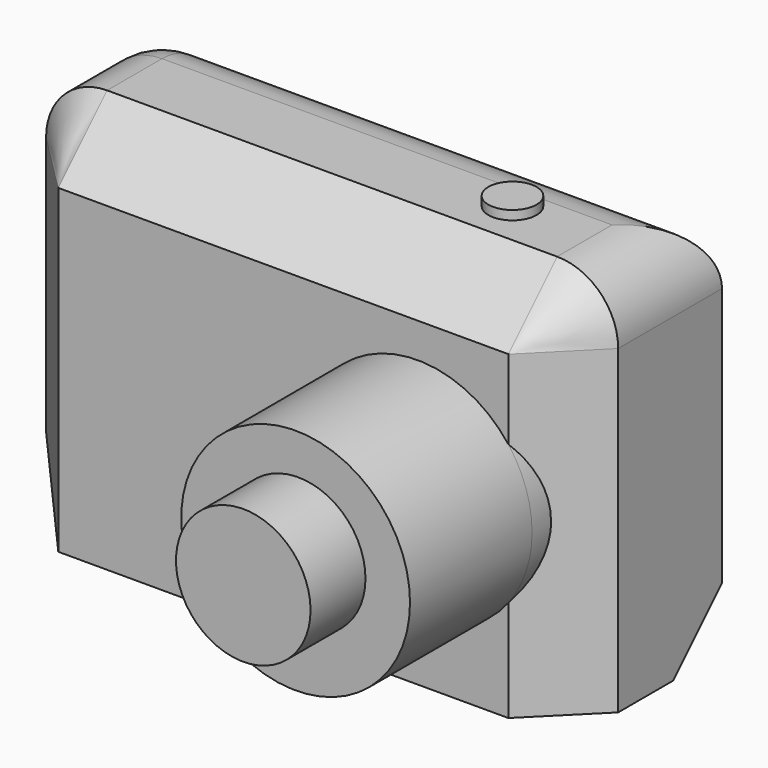
from build123d import *

# Parameters (mm, degrees)
F0_W         = 150
F0_H         = 50
F1_DEPTH     = 100
F2_R         = 30
F3_DEPTH     = 40
F4_R         = 16
F5_R         = 16
F6_T1_DEPTH  = 75.1469278075
F6_T3_DEPTH  = 125.1469278075
F6_T5_DEPTH  = 175.1469278075
F6_T7_DEPTH  = 118
F6_T10_ANGLE = 90
F6_T12_ANGLE = 90
F6_T14_ANGLE = 90
F6_T18_DEPTH = 125.1469278075
F6_S19_R     = 30
F6_T20_DEPTH = 65
F7_R         = 6.3155551437
F8_DEPTH     = 2.4
F9_R         = 17.6407421848
F10_DEPTH    = 18


# Not quite as in the source:
# - a fillet or chamfer that OpenCascade refuses, or shapes differently, is made with other operations: its cross-section is extruded or revolved along the edge and cut away or added


with BuildPart() as f1:
    # F0 (on Top) → F1 (new body)
    with BuildSketch(Plane.XY):
        with Locations((-90.5639529228, -72.1464735391)):
            Rectangle(F0_W, F0_H)
    extrude(amount=F1_DEPTH)

    # F2 (on face) → F3 (join)
    with BuildSketch(Plane.XZ.offset(97.1464735391)):
        with Locations((-55.3404204547, 44.8933616281)):
            Circle(F2_R)
    extrude(amount=F3_DEPTH)

    # F4
    f4_edges = [f1.edges().sort_by_distance(p)[0] for p in [
        (-165.563953, -72.146474, 100),
    ]]
    fillet(f4_edges, radius=F4_R)

    # F5
    f5_edges = [f1.edges().sort_by_distance(p)[0] for p in [
        (-15.563953, -72.146474, 100),
        (-82.563953, -47.146474, 100),
    ]]
    fillet(f5_edges, radius=F5_R)

    # F6: chamfer of 16 on 4 edges, made by hand

    # F6_s2 → F6_t1 (cut)
    with BuildSketch(Plane.XZ.offset(63.1464735391)):
        Polygon((-149.5639529228, 0), (-165.5639529228, 16), (-165.5639529228, 0), align=None)
    extrude(amount=F6_T1_DEPTH, mode=Mode.SUBTRACT)

    # F6_s4 → F6_t3 (cut)
    with BuildSketch(Plane.XY.offset(-41.1469278075)):
        Polygon((-165.5639529228, -81.1464735391), (-149.5639529228, -97.1464735391), (-165.5639529228, -97.1464735391), align=None)
    extrude(amount=F6_T3_DEPTH, mode=Mode.SUBTRACT)

    # F6_s6 → F6_t5 (cut)
    with BuildSketch(Plane.YZ.offset(-149.5639529228)):
        Polygon((-47.1464735391, 16), (-63.1464735391, 0), (-47.1464735391, 0), align=None)
    extrude(amount=F6_T5_DEPTH, mode=Mode.SUBTRACT)

    # F6_s8 → F6_t7 (cut)
    with BuildSketch(Plane.YZ.offset(-149.5639529228)):
        Polygon((-97.1464735391, 84), (-81.1464735391, 100), (-97.1464735391, 100), align=None)
    extrude(amount=F6_T7_DEPTH, mode=Mode.SUBTRACT)

    # F6_s9 → F6_t10 (revolve, cut)
    with BuildSketch(Plane.YZ.offset(-149.5639529228)):
        Polygon((-63.1464735391, 0), (-47.1464735391, 16), (-47.1464735391, 0), align=None)
    revolve(axis=Axis((-149.5639529228, -63.1464735391, 0), (0, 0, 1)), revolution_arc=F6_T10_ANGLE, mode=Mode.SUBTRACT)

    # F6_s11 → F6_t12 (revolve, cut)
    with BuildSketch(Plane.XY.offset(84)):
        Polygon((-149.5639529228, -97.1464735391), (-165.5639529228, -81.1464735391), (-165.5639529228, -97.1464735391), align=None)
    revolve(axis=Axis((-149.5639529228, -97.1464735391, 84), (0, 1, 0)), revolution_arc=F6_T12_ANGLE, mode=Mode.SUBTRACT)

    # F6_s13 → F6_t14 (revolve, cut)
    with BuildSketch(Plane.YZ.offset(-31.5639529228)):
        Polygon((-97.1464735391, 84), (-81.1464735391, 100), (-97.1464735391, 100), align=None)
    revolve(axis=Axis((-31.5639529228, -97.1464735391, 84), (0, 1, 0)), revolution_arc=F6_T14_ANGLE, mode=Mode.SUBTRACT)


with BuildPart() as f6_tool16:
    # F6_s17 → F6_t18 (new body)
    with BuildSketch(Plane.XY.offset(-41.1469278075)):
        Polygon((-15.5639529228, -81.1464735391), (-31.5639529228, -97.1464735391), (-15.5639529228, -97.1464735391), align=None)
    extrude(amount=F6_T18_DEPTH)

    # F6_s19 → F6_t20 (cut, symmetric)
    with BuildSketch(Plane.XZ.offset(89.1)):
        with Locations((-55.3404204547, 44.8933616281)):
            Circle(F6_S19_R)
    extrude(amount=F6_T20_DEPTH, both=True, mode=Mode.SUBTRACT)


with BuildPart() as f1_1:
    add(f1.part)

    # F6_t15: cut F6_tool16
    add(f6_tool16.part, mode=Mode.SUBTRACT)

    # F7 (on face) → F8 (join)
    with BuildSketch(Plane.XY.offset(100)):
        with Locations((-52.6833832264, -69.3942382932)):
            Circle(F7_R)
    extrude(amount=F8_DEPTH)

    # F9 (on face) → F10 (join)
    with BuildSketch(Plane.XZ.offset(137.1464735391)):
        with Locations((-54.6616874635, 46.6945059597)):
            Circle(F9_R)
    extrude(amount=F10_DEPTH)


solid = f1_1.part
